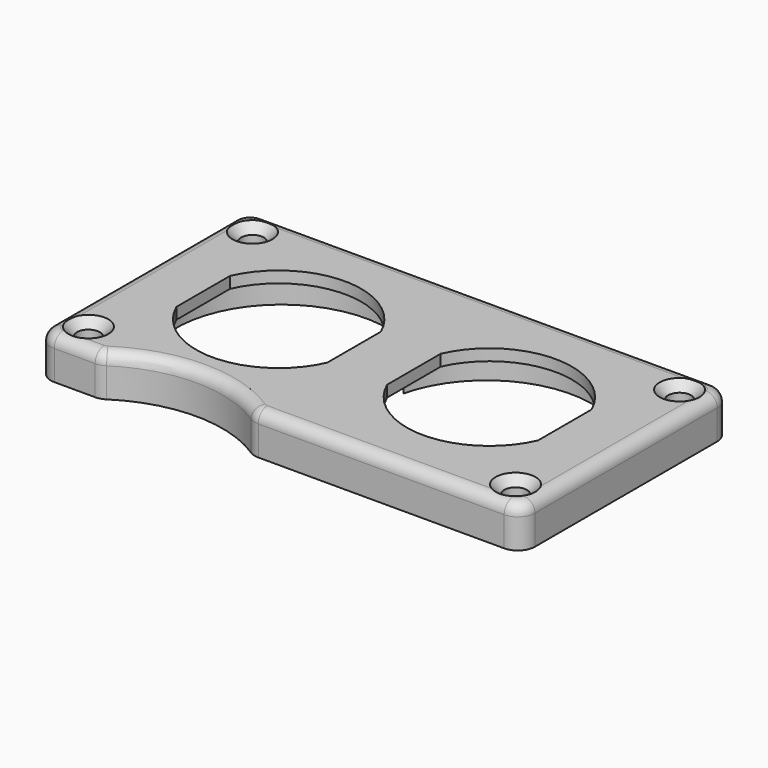
from build123d import *

# Parameters (mm, degrees)
F0_R     = 2
F1_DEPTH = 7.2
F3_DEPTH = 5.2
F4_R     = 2


# Not quite as in the source:
# - a fillet or chamfer that OpenCascade refuses, or shapes differently, is made with other operations: its cross-section is extruded or revolved along the edge and cut away or added
# - a feature names something its author has since deleted; it is built from what else it names


with BuildPart() as f1:
    # F0 (on Top) → F1 (new body)
    with BuildSketch(Plane.XY):
        with BuildLine():
            Line((-3.6799965084, -23), (39.5, -23))
            ThreePointArc((39.5, -23), (41.6213203436, -22.1213203436), (42.5, -20))
            Line((42.5, -20), (42.5, 20))
            ThreePointArc((42.5, 20), (41.6213203436, 22.1213203436), (39.5, 23))
            Line((39.5, 23), (-39.5, 23))
            ThreePointArc((-39.5, 23), (-41.6213203436, 22.1213203436), (-42.5, 20))
            Line((-42.5, 20), (-42.5, 0))
            Line((-42.5, 0), (-42.5, -20))
            ThreePointArc((-42.5, -20), (-41.6213203436, -22.1213203436), (-39.5, -23))
            Line((-39.5, -23), (-32.3200034916, -23))
            ThreePointArc((-32.3200034916, -23), (-31.4664395347, -22.8760091397), (-30.683431664, -22.5142857143))
            ThreePointArc((-30.683431664, -22.5142857143), (-18, -18.75), (-5.316568336, -22.5142857143))
            ThreePointArc((-5.316568336, -22.5142857143), (-4.5335604653, -22.8760091397), (-3.6799965084, -23))
        make_face()
        with Locations((-37.5, -18)):
            Circle(F0_R, mode=Mode.SUBTRACT)
        with Locations((37.5, -18)):
            Circle(F0_R, mode=Mode.SUBTRACT)
        with BuildLine():
            ThreePointArc((-31.75, 5.8896094947), (-18.5, 14.5), (-5.25, 5.8896094947))
            Line((-5.25, 5.8896094947), (-5.25, -5.8896094947))
            ThreePointArc((-5.25, -5.8896094947), (-18.5, -14.5), (-31.75, -5.8896094947))
            Line((-31.75, -5.8896094947), (-31.75, 5.8896094947))
        make_face(mode=Mode.SUBTRACT)
        with Locations((-37.5, 18)):
            Circle(F0_R, mode=Mode.SUBTRACT)
        with BuildLine():
            ThreePointArc((31.75, -5.8896094947), (18.5, -14.5), (5.25, -5.8896094947))
            Line((5.25, -5.8896094947), (5.25, 5.8896094947))
            ThreePointArc((5.25, 5.8896094947), (18.5, 14.5), (31.75, 5.8896094947))
            Line((31.75, 5.8896094947), (31.75, -5.8896094947))
        make_face(mode=Mode.SUBTRACT)
        with Locations((37.5, 18)):
            Circle(F0_R, mode=Mode.SUBTRACT)
    extrude(amount=F1_DEPTH)

    # F2 (on face) → F3 (cut)
    with BuildSketch(Plane(origin=(0, 0, 0), x_dir=(1, 0, 0), z_dir=(0, 0, -1))):
        with BuildLine():
            ThreePointArc((0, 4.2720018727), (-36.5, 0), (0, -4.2720018727))
            ThreePointArc((0, -4.2720018727), (36.5, 0), (0, 4.2720018727))
        make_face()
    extrude(amount=-F3_DEPTH, mode=Mode.SUBTRACT)

    # F4
    f4_edges = [f1.edges().sort_by_distance(p)[0] for p in [
        (0, 23, 7.2),
        (-41.62132, 22.12132, 7.2),
        (-42.5, 0, 7.2),
        (-41.62132, -22.12132, 7.2),
        (-35.910002, -23, 7.2),
        (17.910002, -23, 7.2),
        (41.62132, -22.12132, 7.2),
        (42.5, 0, 7.2),
        (41.62132, 22.12132, 7.2),
        (-18, -18.75, 7.2),
        (-31.46644, -22.876009, 7.2),
        (-4.53356, -22.876009, 7.2),
    ]]
    fillet(f4_edges, radius=F4_R)

    # F5: chamfer of 1.5 on 4 edges, made by hand

    # F5_s1 → F5_t2 (revolve, cut)
    with BuildSketch(Plane.XZ.offset(-18)):
        Polygon((-34, 7.2), (-35.5, 5.7), (-35.5, 7.2), align=None)
    revolve(axis=Axis((-37.5, 18, 7.2), (0, 0, 1)), mode=Mode.SUBTRACT)

    # F5_s3 → F5_t4 (revolve, cut)
    with BuildSketch(Plane.XZ.offset(18)):
        Polygon((-34, 7.2), (-35.5, 5.7), (-35.5, 7.2), align=None)
    revolve(axis=Axis((-37.5, -18, 7.2), (0, 0, 1)), mode=Mode.SUBTRACT)

    # F5_s5 → F5_t6 (revolve, cut)
    with BuildSketch(Plane.XZ.offset(18)):
        Polygon((41, 7.2), (39.5, 5.7), (39.5, 7.2), align=None)
    revolve(axis=Axis((37.5, -18, 7.2), (0, 0, 1)), mode=Mode.SUBTRACT)

    # F5_s7 → F5_t8 (revolve, cut)
    with BuildSketch(Plane.XZ.offset(-18)):
        Polygon((41, 7.2), (39.5, 5.7), (39.5, 7.2), align=None)
    revolve(axis=Axis((37.5, 18, 7.2), (0, 0, 1)), mode=Mode.SUBTRACT)


solid = f1.part
